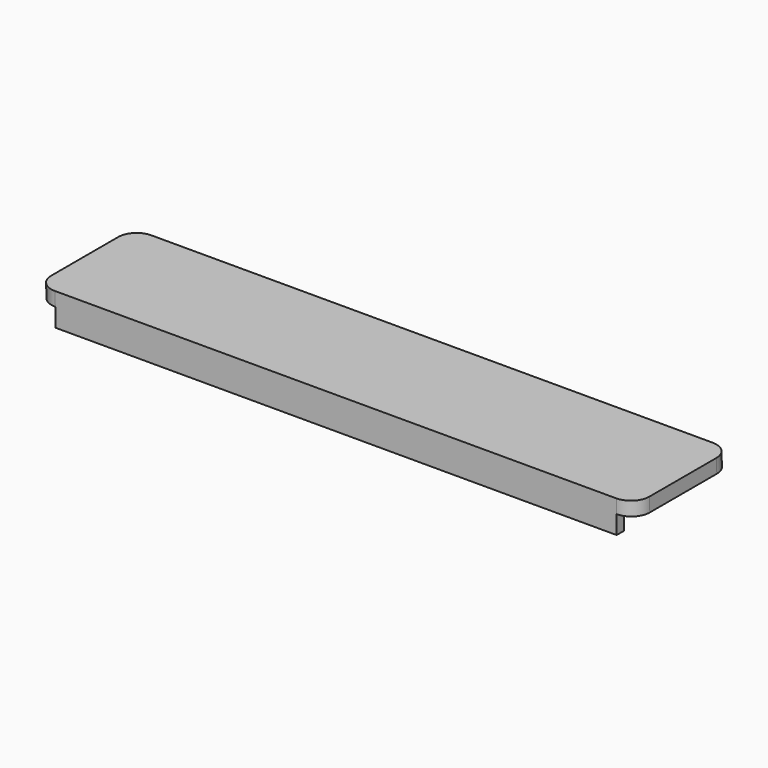
from build123d import *

# Parameters (mm, degrees)
F1_DEPTH = 13.1
F3_R     = 2
F2_W     = 61
F2_H     = 1
F4_DEPTH = 2


# Not quite as in the source:
# - a feature names something its author has since deleted; it is built from what else it names


with BuildPart() as f1:
    # F0 (on Front) → F1 (new body)
    with BuildSketch(Plane.XZ):
        Polygon((22.7466161251, 39.9272560477), (-42.2533838749, 39.9272560477), (-42.2077284126, 38.4279510158), (22.7922715837, 38.4272560477), align=None)
    extrude(amount=F1_DEPTH)

    # F3
    f3_edges = [f1.edges().sort_by_distance(p)[0] for p in [
        (-42.230556, -13.1, 39.177604),
        (22.769444, -13.1, 39.177256),
        (22.769444, 0, 39.177256),
        (-42.230556, 0, 39.177604),
    ]]
    fillet(f3_edges, radius=F3_R)

    # F2 (on face) → F4 (join)
    with BuildSketch(Plane(origin=(0.0004108598, 0, 38.4274997341), x_dir=(0.9999999999, 0, -1.06918e-05), z_dir=(-1.06918e-05, 0, -0.9999999999))):
        with Locations((-9.7081392748, 12.6)):
            Rectangle(F2_W, F2_H)
    extrude(amount=F4_DEPTH)


solid = f1.part
